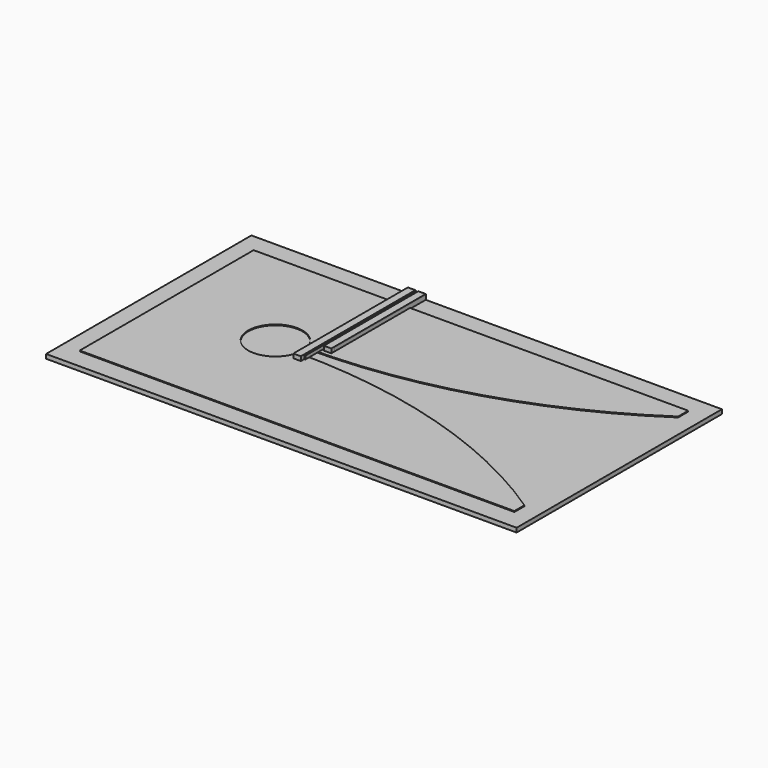
from build123d import *

# Parameters (mm, degrees)
F1_DEPTH  = 0.2
F2_W      = 110
F2_H      = 60
F3_DEPTH  = 1
F5_DEPTH  = 0.8
F6_W      = 4.1765728965
F6_H      = 4.6
F7_DEPTH  = 1
F8_W      = 1.75
F8_H      = 32.4733061887
F9_DEPTH  = 0.2
F8_H_2    = 26.6
F10_W     = 1.75
F10_H     = 1
F11_DEPTH = 1


with BuildPart() as f1:
    # F0 (on Top) → F1 (new body)
    with BuildSketch(Plane.XY):
        with BuildLine():
            Line((-50.8, 25.4), (-50.8, 0))
            Line((-50.8, 0), (-31.75, 0))
            ThreePointArc((-31.75, 0), (-26.0382651501, 6.3178412134), (-19.1783094179, 1.2700654709))
            ThreePointArc((-19.1783094179, 1.2700654709), (17.3850333876, 6.6649625336), (50.8, 22.4580926135))
            Line((50.8, 22.4580926135), (50.8, 25.4))
            Line((50.8, 25.4), (-50.8, 25.4))
        make_face()
        with BuildLine():
            Line((-50.8, -25.4), (50.8, -25.4))
            Line((50.8, -25.4), (50.8, -22.4580926135))
            ThreePointArc((50.8, -22.4580926135), (17.3850333876, -6.6649625336), (-19.1783094179, -1.2700654709))
            ThreePointArc((-19.1783094179, -1.2700654709), (-26.0382651501, -6.3178412134), (-31.75, 0))
            Line((-31.75, 0), (-50.8, 0))
            Line((-50.8, 0), (-50.8, -25.4))
        make_face()
    extrude(amount=F1_DEPTH)



with BuildPart() as f3:
    # F2 (on face) → F3 (new body)
    with BuildSketch(Plane(origin=(0, 0, 0), x_dir=(1, 0, 0), z_dir=(0, 0, -1))):
        Rectangle(F2_W, F2_H)
        with BuildLine():
            Line((-50.8, -25.4), (-50.8, 25.4))
            Line((-50.8, 25.4), (50.8, 25.4))
            Line((50.8, 25.4), (50.8, 22.4580926135))
            ThreePointArc((50.8, 22.4580926135), (17.3850333876, 6.6649625336), (-19.1783094179, 1.2700654709))
            ThreePointArc((-19.1783094179, 1.2700654709), (-31.75, 0), (-19.1783094179, -1.2700654709))
            ThreePointArc((-19.1783094179, -1.2700654709), (17.3850333876, -6.6649625336), (50.8, -22.4580926135))
            Line((50.8, -22.4580926135), (50.8, -25.4))
            Line((50.8, -25.4), (-50.8, -25.4))
        make_face(mode=Mode.SUBTRACT)
        with BuildLine():
            Line((50.8, 25.4), (-50.8, 25.4))
            Line((-50.8, 25.4), (-50.8, -25.4))
            Line((-50.8, -25.4), (50.8, -25.4))
            Line((50.8, -25.4), (50.8, -22.4580926135))
            ThreePointArc((50.8, -22.4580926135), (17.3850333876, -6.6649625336), (-19.1783094179, -1.2700654709))
            ThreePointArc((-19.1783094179, -1.2700654709), (-31.75, 0), (-19.1783094179, 1.2700654709))
            ThreePointArc((-19.1783094179, 1.2700654709), (17.3850333876, 6.6649625336), (50.8, 22.4580926135))
            Line((50.8, 22.4580926135), (50.8, 25.4))
        make_face()
    extrude(amount=F3_DEPTH)



with BuildPart() as f5:
    # F4 (on face) → F5 (new body)
    with BuildSketch(Plane.XY.offset(0.2)):
        with BuildLine():
            ThreePointArc((-16.4155218303, -1.2976037429), (-17.4154701214, -1.2806251524), (-18.4155218303, -1.2716009111))
            Line((-18.4155218303, -1.2716009111), (-18.4155218303, -2.4733061887))
            Line((-18.4155218303, -2.4733061887), (-16.4155218303, -2.4733061887))
            Line((-16.4155218303, -2.4733061887), (-16.4155218303, -1.2976037429))
        make_face()
        with BuildLine():
            ThreePointArc((-16.4155218303, 1.2976037429), (-17.4154701214, 1.2806251524), (-18.4155218303, 1.2716009111))
            Line((-18.4155218303, 1.2716009111), (-18.4155218303, -1.2716009111))
            ThreePointArc((-18.4155218303, -1.2716009111), (-17.4154701214, -1.2806251524), (-16.4155218303, -1.2976037429))
            Line((-16.4155218303, -1.2976037429), (-16.4155218303, 1.2976037429))
        make_face()
        with BuildLine():
            Line((-16.4155218303, 3.4), (-18.4155218303, 3.4))
            Line((-18.4155218303, 3.4), (-18.4155218303, 1.2716009111))
            ThreePointArc((-18.4155218303, 1.2716009111), (-17.4154701214, 1.2806251524), (-16.4155218303, 1.2976037429))
            Line((-16.4155218303, 1.2976037429), (-16.4155218303, 3.4))
        make_face()
        Polygon((-18.4155218303, 25.4), (-18.4155218303, 3.4), (-16.4155218303, 3.4), (-14.2389489338, 3.4), (-14.2389489338, 25.4), align=None)
    extrude(amount=F5_DEPTH)


with BuildPart() as f3_1:
    add(f3.part)

    add(f5.part)  # F7 merges F5
    # F6 (on face) → F7 (join)
    with BuildSketch(Plane.XY):
        with Locations((-16.3272353821, 27.7)):
            Rectangle(F6_W, F6_H)
    extrude(amount=F7_DEPTH)


with BuildPart() as f9:
    # F8 (on face) → F9 (new body)
    with BuildSketch(Plane.XY.offset(1)):
        with Locations((-17.5405218303, 13.7633469056)):
            Rectangle(F8_W, F8_H)
    extrude(amount=F9_DEPTH)


with BuildPart() as f9b:
    # F8 (on face) → F9, piece 2 (new body)
    with BuildSketch(Plane.XY.offset(1)):
        with Locations((-15.1139489338, 16.7)):
            Rectangle(F8_W, F8_H_2)
    extrude(amount=F9_DEPTH)


with BuildPart() as f1_1:
    add(f1.part)

    add(f9.part)  # F11 merges F9

    add(f9b.part)  # F11 merges F9b
    # F10 (on face) → F11 (join)
    with BuildSketch(Plane.XY.offset(0.2)):
        with Locations((-17.5405218303, -2.9733061887)):
            Rectangle(F10_W, F10_H)
        with Locations((-15.1139489338, 2.9)):
            Rectangle(F10_W, F10_H)
    extrude(amount=F11_DEPTH)


solid = Compound([f3_1.part, f1_1.part])
